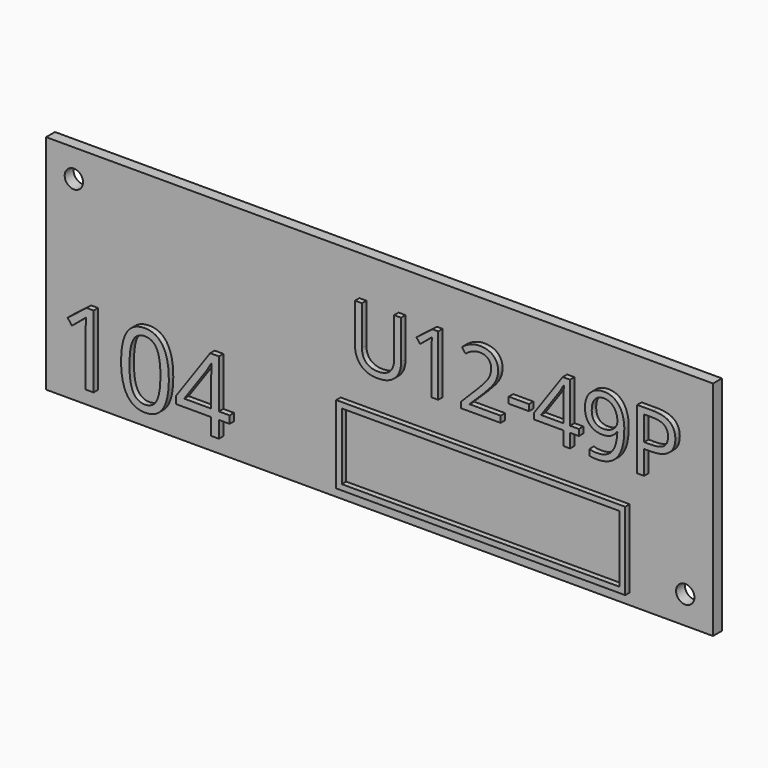
from build123d import *

# Parameters (mm, degrees)
F0_W         = 120
F0_H         = 40
F1_DEPTH     = 2
F3_D         = 3.3
F4_TEXT_SIZE = 15.1814659603
F5_DEPTH     = 1
F6_TEXT_SIZE = 18.1818181818
F7_DEPTH     = 1
F8_W         = 52
F8_H         = 14
F8_W_2       = 49.99999962
F8_H_2       = 11.99999962
F9_DEPTH     = 1


# Not quite as in the source:
# - Text() gives the source's letters only with a copy of the font that has no kerning and outlines rounded to 1/6400 em; it was checked with that copy


with BuildPart() as f1:
    # F0 (on Front) → F1 (new body)
    with BuildSketch(Plane.XZ):
        Rectangle(F0_W, F0_H)
    extrude(amount=F1_DEPTH)

    # F3 (through all)
    with Locations(Plane.XZ.offset(2)):
        with Locations((-55, 15), (55, -15)):
            Hole(F3_D / 2)

    # F4 (on face) → F5 (join)
    with BuildSketch(Plane.XZ.offset(2)):
        with Locations((-5, 2)):
            Text('U12-49P', F4_TEXT_SIZE, font='Open Sans', text_align=(TextAlign.LEFT, TextAlign.BOTTOM))
    extrude(amount=F5_DEPTH)

    # F6 (on face) → F7 (join)
    with BuildSketch(Plane.XZ.offset(2)):
        with Locations((-57, -17)):
            Text('104', F6_TEXT_SIZE, font='Open Sans', text_align=(TextAlign.LEFT, TextAlign.BOTTOM))
    extrude(amount=F7_DEPTH)

    # F8 (on face) → F9 (join)
    with BuildSketch(Plane.XZ.offset(2)):
        with Locations((19, -11)):
            Rectangle(F8_W, F8_H)
        with Locations((19, -11)):
            Rectangle(F8_W_2, F8_H_2, mode=Mode.SUBTRACT)
    extrude(amount=F9_DEPTH)


solid = f1.part
